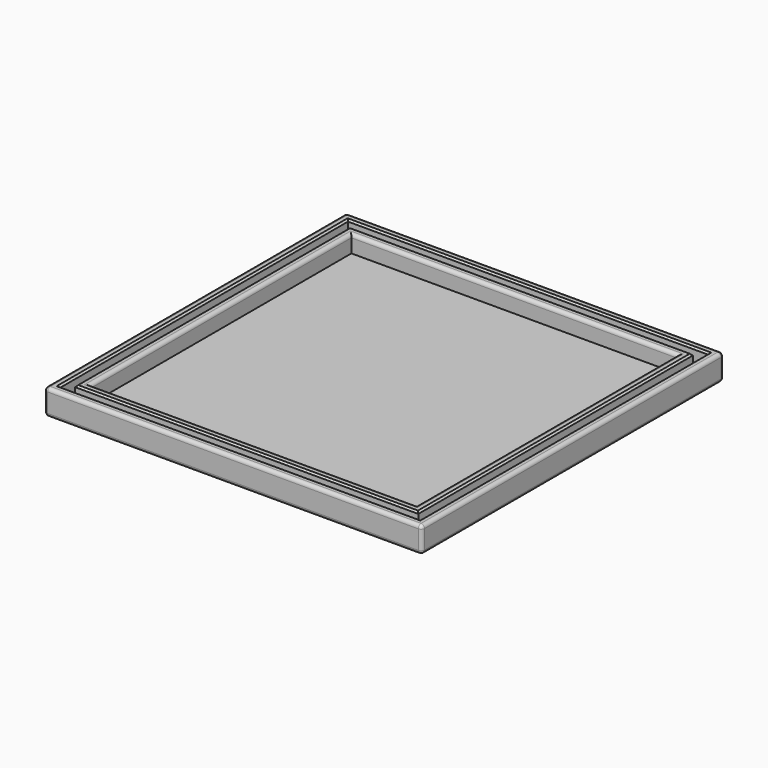
from build123d import *

# Parameters (mm, degrees)
F0_W         = 279.4
F0_H         = 279.4
F0_W_2       = 266.7
F0_H_2       = 266.7
F0_W_3       = 254
F0_H_3       = 254
F0_W_4       = 241.3
F0_H_4       = 241.3
F1_DEPTH     = 6.35
F2_DEPTH     = 19.05
F3_SIZE      = 1.27
F4_R         = 2.54
F5_T1_DEPTH  = 274.32
F5_T3_DEPTH  = 274.32
F5_T5_DEPTH  = 13.97
F5_S9_W      = 2.54
F5_S9_H      = 2.54
F5_T10_DEPTH = 2.54
F5_S15_W     = 2.54
F5_S15_H     = 2.54
F5_T16_DEPTH = 2.54
F5_S21_W     = 2.54
F5_S21_H     = 2.54
F5_T22_DEPTH = 2.54
F5_S27_W     = 2.54
F5_S27_H     = 2.54
F5_T28_DEPTH = 2.54
F5_S33_W     = 2.54
F5_S33_H     = 2.54
F5_T34_DEPTH = 2.54
F5_S39_W     = 2.54
F5_S39_H     = 2.54
F5_T40_DEPTH = 2.54
F5_S45_W     = 2.54
F5_S45_H     = 2.54
F5_T46_DEPTH = 2.54
F5_S51_W     = 2.54
F5_S51_H     = 2.54
F5_T52_DEPTH = 2.54


# Not quite as in the source:
# - a fillet or chamfer that OpenCascade refuses, or shapes differently, is made with other operations: its cross-section is extruded or revolved along the edge and cut away or added


with BuildPart() as f1:
    # F0 (on Top) → F1 (new body)
    with BuildSketch(Plane.XY):
        Rectangle(F0_W, F0_H)
        Rectangle(F0_W_2, F0_H_2, mode=Mode.SUBTRACT)
        Rectangle(F0_W_2, F0_H_2)
        Rectangle(F0_W_3, F0_H_3, mode=Mode.SUBTRACT)
        Rectangle(F0_W_3, F0_H_3)
        Rectangle(F0_W_4, F0_H_4, mode=Mode.SUBTRACT)
        Rectangle(F0_W_4, F0_H_4)
    extrude(amount=F1_DEPTH)

    # F0 (on Top) → F2 (join)
    with BuildSketch(Plane.XY):
        Rectangle(F0_W, F0_H)
        Rectangle(F0_W_2, F0_H_2, mode=Mode.SUBTRACT)
        Rectangle(F0_W_3, F0_H_3)
        Rectangle(F0_W_4, F0_H_4, mode=Mode.SUBTRACT)
    extrude(amount=F2_DEPTH)

    # F3
    f3_edges = [f1.edges().sort_by_distance(p)[0] for p in [
        (-127, 0, 19.05),
        (-133.35, 0, 19.05),
        (0, 133.35, 19.05),
        (0, 127, 19.05),
        (133.35, 0, 19.05),
        (127, 0, 19.05),
        (0, -127, 19.05),
        (0, -133.35, 19.05),
    ]]
    chamfer(f3_edges, length=F3_SIZE)

    # F4
    f4_edges = [f1.edges().sort_by_distance(p)[0] for p in [
        (-139.7, 0, 19.05),
        (0, 139.7, 19.05),
        (139.7, 0, 19.05),
        (0, -139.7, 19.05),
        (-120.65, 0, 19.05),
        (0, -120.65, 19.05),
        (120.65, 0, 19.05),
        (0, 120.65, 19.05),
    ]]
    fillet(f4_edges, radius=F4_R)

    # F5: fillet of radius 2.54 on 8 edges, made by hand

    # F5_s2 → F5_t1 (cut)
    with BuildSketch(Plane.YZ.offset(-137.16)):
        with BuildLine():
            ThreePointArc((139.7, 2.54), (138.9560512242, 0.7439487758), (137.16, 0))
            Line((137.16, 0), (139.7, 0))
            Line((139.7, 0), (139.7, 2.54))
        make_face()
        with BuildLine():
            ThreePointArc((-139.7, 2.54), (-138.9560512242, 0.7439487758), (-137.16, 0))
            Line((-137.16, 0), (-139.7, 0))
            Line((-139.7, 0), (-139.7, 2.54))
        make_face()
    extrude(amount=F5_T1_DEPTH, mode=Mode.SUBTRACT)

    # F5_s4 → F5_t3 (cut)
    with BuildSketch(Plane.XZ.offset(-137.16)):
        with BuildLine():
            ThreePointArc((-139.7, 2.54), (-138.9560512242, 0.7439487758), (-137.16, 0))
            Line((-137.16, 0), (-139.7, 0))
            Line((-139.7, 0), (-139.7, 2.54))
        make_face()
        with BuildLine():
            ThreePointArc((139.7, 2.54), (138.9560512242, 0.7439487758), (137.16, 0))
            Line((137.16, 0), (139.7, 0))
            Line((139.7, 0), (139.7, 2.54))
        make_face()
    extrude(amount=F5_T3_DEPTH, mode=Mode.SUBTRACT)

    # F5_s6 → F5_t5 (cut)
    with BuildSketch(Plane.XY.offset(2.54)):
        with BuildLine():
            ThreePointArc((137.16, 139.7), (138.9560512242, 138.9560512242), (139.7, 137.16))
            Line((139.7, 137.16), (139.7, 139.7))
            Line((139.7, 139.7), (137.16, 139.7))
        make_face()
        with BuildLine():
            ThreePointArc((-139.7, 137.16), (-138.9560512242, 138.9560512242), (-137.16, 139.7))
            Line((-137.16, 139.7), (-139.7, 139.7))
            Line((-139.7, 139.7), (-139.7, 137.16))
        make_face()
        with BuildLine():
            ThreePointArc((-139.7, -137.16), (-138.9560512242, -138.9560512242), (-137.16, -139.7))
            Line((-137.16, -139.7), (-139.7, -139.7))
            Line((-139.7, -139.7), (-139.7, -137.16))
        make_face()
        with BuildLine():
            ThreePointArc((137.16, -139.7), (138.9560512242, -138.9560512242), (139.7, -137.16))
            Line((139.7, -137.16), (139.7, -139.7))
            Line((139.7, -139.7), (137.16, -139.7))
        make_face()
    extrude(amount=F5_T5_DEPTH, mode=Mode.SUBTRACT)


with BuildPart() as f5_tool8:
    # F5_s9 → F5_t10 (new body)
    with BuildSketch(Plane.XZ.offset(137.16)):
        with Locations((138.43, 17.78)):
            Rectangle(F5_S9_W, F5_S9_H)
    extrude(amount=F5_T10_DEPTH)

    # F5_s11 → F5_t12 (revolve, cut)
    with BuildSketch(Plane(origin=(137.16, -137.16, 16.51), x_dir=(-0.7071067812, 0, -0.7071067812), z_dir=(-0.7071067812, 0, 0.7071067812))):
        with BuildLine():
            ThreePointArc((0, -2.54), (2.54, 0), (0, 2.54))
            Line((0, 2.54), (0, -2.54))
        make_face()
    revolve(axis=Axis((137.16, -137.16, 16.51), (0, -1, 0)), mode=Mode.SUBTRACT)


with BuildPart() as f1_1:
    add(f1.part)

    # F5_t7: cut F5_tool8
    add(f5_tool8.part, mode=Mode.SUBTRACT)


with BuildPart() as f5_tool14:
    # F5_s15 → F5_t16 (new body)
    with BuildSketch(Plane.YZ.offset(-137.16)):
        with Locations((-138.43, 17.78)):
            Rectangle(F5_S15_W, F5_S15_H)
    extrude(amount=-F5_T16_DEPTH)

    # F5_s17 → F5_t18 (revolve, cut)
    with BuildSketch(Plane(origin=(-137.16, -137.16, 16.51), x_dir=(0, 0.7071067812, -0.7071067812), z_dir=(0, 0.7071067812, 0.7071067812))):
        with BuildLine():
            ThreePointArc((0, -2.54), (2.54, 0), (0, 2.54))
            Line((0, 2.54), (0, -2.54))
        make_face()
    revolve(axis=Axis((-137.16, -137.16, 16.51), (-1, 0, 0)), mode=Mode.SUBTRACT)


with BuildPart() as f1_2:
    add(f1_1.part)

    # F5_t13: cut F5_tool14
    add(f5_tool14.part, mode=Mode.SUBTRACT)


with BuildPart() as f5_tool20:
    # F5_s21 → F5_t22 (new body)
    with BuildSketch(Plane.YZ.offset(-137.16)):
        with Locations((138.43, 17.78)):
            Rectangle(F5_S21_W, F5_S21_H)
    extrude(amount=-F5_T22_DEPTH)

    # F5_s23 → F5_t24 (revolve, cut)
    with BuildSketch(Plane(origin=(-137.16, 137.16, 16.51), x_dir=(0, -0.7071067812, -0.7071067812), z_dir=(0, 0.7071067812, -0.7071067812))):
        with BuildLine():
            ThreePointArc((0, -2.54), (2.54, 0), (0, 2.54))
            Line((0, 2.54), (0, -2.54))
        make_face()
    revolve(axis=Axis((-137.16, 137.16, 16.51), (-1, 0, 0)), mode=Mode.SUBTRACT)


with BuildPart() as f1_3:
    add(f1_2.part)

    # F5_t19: cut F5_tool20
    add(f5_tool20.part, mode=Mode.SUBTRACT)


with BuildPart() as f5_tool26:
    # F5_s27 → F5_t28 (new body)
    with BuildSketch(Plane.XZ.offset(-137.16)):
        with Locations((138.43, 17.78)):
            Rectangle(F5_S27_W, F5_S27_H)
    extrude(amount=-F5_T28_DEPTH)

    # F5_s29 → F5_t30 (revolve, cut)
    with BuildSketch(Plane(origin=(137.16, 137.16, 16.51), x_dir=(-0.7071067812, 0, -0.7071067812), z_dir=(0.7071067812, 0, -0.7071067812))):
        with BuildLine():
            ThreePointArc((0, -2.54), (2.54, 0), (0, 2.54))
            Line((0, 2.54), (0, -2.54))
        make_face()
    revolve(axis=Axis((137.16, 137.16, 16.51), (0, 1, 0)), mode=Mode.SUBTRACT)


with BuildPart() as f1_4:
    add(f1_3.part)

    # F5_t25: cut F5_tool26
    add(f5_tool26.part, mode=Mode.SUBTRACT)


with BuildPart() as f5_tool32:
    # F5_s33 → F5_t34 (new body)
    with BuildSketch(Plane.XY.offset(2.54)):
        with Locations((138.43, 138.43)):
            Rectangle(F5_S33_W, F5_S33_H)
    extrude(amount=-F5_T34_DEPTH)

    # F5_s35 → F5_t36 (revolve, cut)
    with BuildSketch(Plane(origin=(137.16, 137.16, 2.54), x_dir=(-0.7071067812, -0.7071067812, 0), z_dir=(0.7071067812, -0.7071067812, 0))):
        with BuildLine():
            ThreePointArc((0, -2.54), (2.54, 0), (0, 2.54))
            Line((0, 2.54), (0, -2.54))
        make_face()
    revolve(axis=Axis((137.16, 137.16, 2.54), (0, 0, -1)), mode=Mode.SUBTRACT)


with BuildPart() as f1_5:
    add(f1_4.part)

    # F5_t31: cut F5_tool32
    add(f5_tool32.part, mode=Mode.SUBTRACT)


with BuildPart() as f5_tool38:
    # F5_s39 → F5_t40 (new body)
    with BuildSketch(Plane.XY.offset(2.54)):
        with Locations((-138.43, 138.43)):
            Rectangle(F5_S39_W, F5_S39_H)
    extrude(amount=-F5_T40_DEPTH)

    # F5_s41 → F5_t42 (revolve, cut)
    with BuildSketch(Plane(origin=(-137.16, 137.16, 2.54), x_dir=(0.7071067812, -0.7071067812, 0), z_dir=(0.7071067812, 0.7071067812, 0))):
        with BuildLine():
            ThreePointArc((0, -2.54), (2.54, 0), (0, 2.54))
            Line((0, 2.54), (0, -2.54))
        make_face()
    revolve(axis=Axis((-137.16, 137.16, 2.54), (0, 0, -1)), mode=Mode.SUBTRACT)


with BuildPart() as f1_6:
    add(f1_5.part)

    # F5_t37: cut F5_tool38
    add(f5_tool38.part, mode=Mode.SUBTRACT)


with BuildPart() as f5_tool44:
    # F5_s45 → F5_t46 (new body)
    with BuildSketch(Plane.YZ.offset(-137.16)):
        with Locations((-138.43, 1.27)):
            Rectangle(F5_S45_W, F5_S45_H)
    extrude(amount=-F5_T46_DEPTH)

    # F5_s47 → F5_t48 (revolve, cut)
    with BuildSketch(Plane(origin=(-137.16, -137.16, 2.54), x_dir=(0, 0.7071067812, 0.7071067812), z_dir=(0, -0.7071067812, 0.7071067812))):
        with BuildLine():
            ThreePointArc((0, -2.54), (2.54, 0), (0, 2.54))
            Line((0, 2.54), (0, -2.54))
        make_face()
    revolve(axis=Axis((-137.16, -137.16, 2.54), (-1, 0, 0)), mode=Mode.SUBTRACT)


with BuildPart() as f1_7:
    add(f1_6.part)

    # F5_t43: cut F5_tool44
    add(f5_tool44.part, mode=Mode.SUBTRACT)


with BuildPart() as f5_tool50:
    # F5_s51 → F5_t52 (new body)
    with BuildSketch(Plane.XY.offset(2.54)):
        with Locations((138.43, -138.43)):
            Rectangle(F5_S51_W, F5_S51_H)
    extrude(amount=-F5_T52_DEPTH)

    # F5_s53 → F5_t54 (revolve, cut)
    with BuildSketch(Plane(origin=(137.16, -137.16, 2.54), x_dir=(-0.7071067812, 0.7071067812, 0), z_dir=(-0.7071067812, -0.7071067812, 0))):
        with BuildLine():
            ThreePointArc((0, -2.54), (2.54, 0), (0, 2.54))
            Line((0, 2.54), (0, -2.54))
        make_face()
    revolve(axis=Axis((137.16, -137.16, 2.54), (0, 0, -1)), mode=Mode.SUBTRACT)


with BuildPart() as f1_8:
    add(f1_7.part)

    # F5_t49: cut F5_tool50
    add(f5_tool50.part, mode=Mode.SUBTRACT)


solid = f1_8.part
